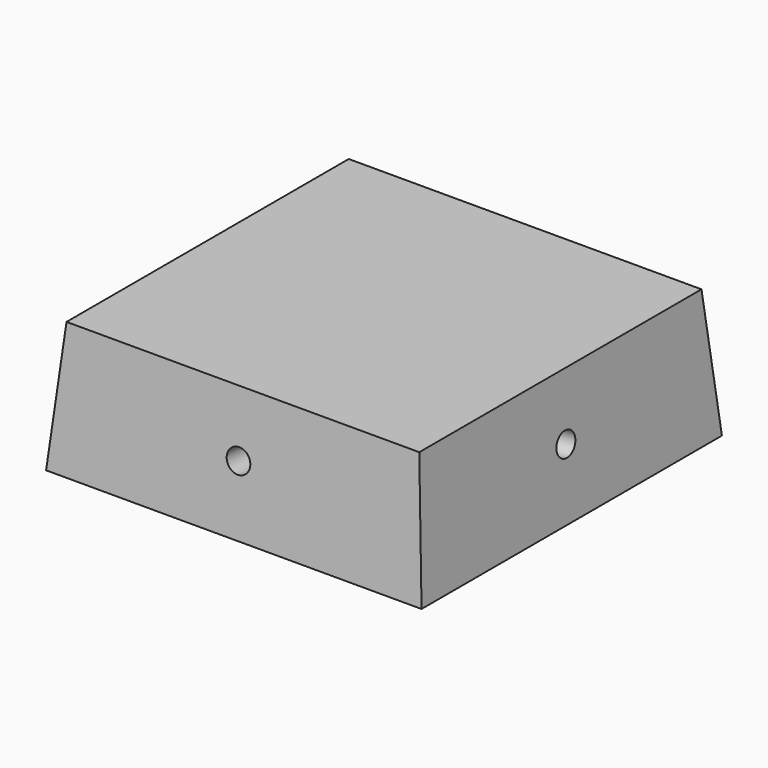
from build123d import *

# Parameters (mm, degrees)
F0_W        = 101.6
F0_H        = 101.6
F1_DEPTH    = 34.925
F2_T1_DEPTH = 299.3404177556
F2_T3_DEPTH = 299.3404177556
F3_R        = 3.175
F4_DEPTH    = 12.7
F5_R        = 3.175
F6_DEPTH    = 12.7
F7_R        = 3.175
F8_DEPTH    = 12.7
F9_R        = 3.175
F10_DEPTH   = 12.7
F11_W       = 75.6562831473
F11_H       = 25.4
F12_DEPTH   = 25.4
F13_SIZE2   = 2.53999
F13_SIZE    = 25.39999


# Not quite as in the source:
# - a fillet or chamfer that OpenCascade refuses, or shapes differently, is made with other operations: its cross-section is extruded or revolved along the edge and cut away or added
# - a fillet or chamfer is up to 0.001 mm smaller than in the source, because OpenCascade refuses the exact size


with BuildPart() as f1:
    # F0 (on Top) → F1 (new body)
    with BuildSketch(Plane.XY):
        Rectangle(F0_W, F0_H)
    extrude(amount=F1_DEPTH)

    # F2: chamfer of 3.3274 x 38.0323560322 on 4 edges, made by hand

    # F2_s2 → F2_t1 (cut)
    with BuildSketch(Plane.XZ.offset(-149.6702088778)):
        Polygon((-50.8, -3.1073560322), (-47.4726, 34.925), (-50.8, 34.925), align=None)
        Polygon((50.8, -3.1073560322), (47.4726, 34.925), (50.8, 34.925), align=None)
    extrude(amount=F2_T1_DEPTH, mode=Mode.SUBTRACT)

    # F2_s4 → F2_t3 (cut)
    with BuildSketch(Plane.YZ.offset(-149.6702088778)):
        Polygon((-50.8, -3.1073560322), (-47.4726, 34.925), (-50.8, 34.925), align=None)
        Polygon((50.8, -3.1073560322), (47.4726, 34.925), (50.8, 34.925), align=None)
    extrude(amount=F2_T3_DEPTH, mode=Mode.SUBTRACT)

    # F3 (on face) → F4 (cut)
    with BuildSketch(Plane(origin=(0, 50.1443235703, 4.3870598526), x_dir=(-1, 0, 0), z_dir=(0, 0.9961946981, 0.0871557427))):
        with Locations((0, 13.6719250414)):
            Circle(F3_R)
    extrude(amount=-F4_DEPTH, mode=Mode.SUBTRACT)

    # F5 (on face) → F6 (cut)
    with BuildSketch(Plane(origin=(0, -50.1443235703, 4.3870598526), x_dir=(1, 0, 0), z_dir=(0, -0.9961946981, 0.0871557427))):
        with Locations((0, 13.6719250414)):
            Circle(F5_R)
    extrude(amount=-F6_DEPTH, mode=Mode.SUBTRACT)

    # F7 (on face) → F8 (cut)
    with BuildSketch(Plane(origin=(50.1443235703, 0, 4.3870598526), x_dir=(0, 1, 0), z_dir=(0.9961946981, 0, 0.0871557427))):
        with Locations((0, 13.6719250414)):
            Circle(F7_R)
    extrude(amount=-F8_DEPTH, mode=Mode.SUBTRACT)

    # F9 (on face) → F10 (cut)
    with BuildSketch(Plane(origin=(-50.1443235703, 0, 4.3870598526), x_dir=(0, -1, 0), z_dir=(-0.9961946981, 0, 0.0871557427))):
        with Locations((0, 13.6719250414)):
            Circle(F9_R)
    extrude(amount=-F10_DEPTH, mode=Mode.SUBTRACT)

    # F11 (on face) → F12 (cut)
    with BuildSketch(Plane(origin=(0, 0, 0), x_dir=(1, 0, 0), z_dir=(0, 0, -1))):
        with Locations((0, -18.7781415736)):
            Rectangle(F11_W, F11_H)
    extrude(amount=-F12_DEPTH, mode=Mode.SUBTRACT)

    # F13 (size 25.4 and 2.54 in the source; OpenCascade refuses exactly that, so slightly less here)
    f13_edges = [f1.edges().sort_by_distance(p)[0] for p in [
        (0, 6.078142, 25.4),
        (-37.828142, 18.778142, 25.4),
        (37.828142, 18.778142, 25.4),
        (0, 31.478142, 25.4),
    ]]
    chamfer(f13_edges, length=F13_SIZE, length2=F13_SIZE2)


solid = f1.part
